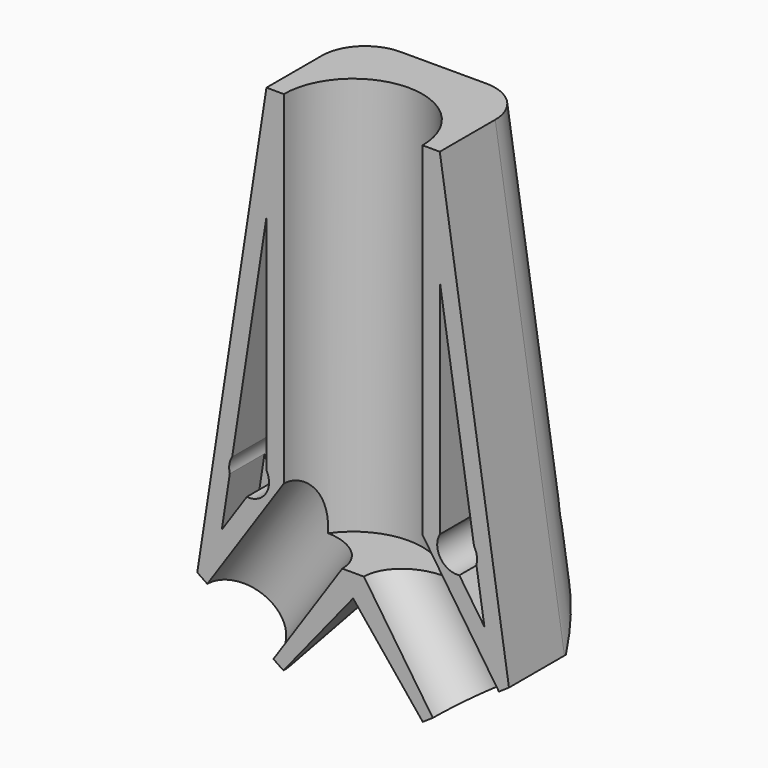
from build123d import *

# Parameters (mm, degrees)
F0_R          = 2.3
F1_DEPTH      = 13
F3_DEPTH      = 46
F6_DEPTH      = 52.2
F8_DEPTH      = 25
F10_DEPTH     = 25
F11_T1_DEPTH  = 69.4664340584
F11_T3_DEPTH  = 69.4664340584
F11_T8_DEPTH  = 31.9524083705
F11_T13_DEPTH = 31.9524083705
F11_T19_DEPTH = 31.9524083705
F11_T23_DEPTH = 31.9524083705
F15_DEPTH     = 5
F16_DEPTH     = 5
F18_R         = 3.2
F19_DEPTH     = 28


# Not quite as in the source:
# - a fillet or chamfer that OpenCascade refuses, or shapes differently, is made with other operations: its cross-section is extruded or revolved along the edge and cut away or added
# - a feature names something its author has since deleted; it is built from what else it names


with BuildPart() as f1:
    # F0 (on Front) → F1 (new body)
    with BuildSketch(Plane.XZ):
        Polygon((10, 40), (-10, 40), (-17.9806351662, -11.8325809017), (-8.0368565166, -18.5498173996), (0, -8.6111112242), (8.0368565166, -18.5498173996), (17.9806351662, -11.8325809017), align=None)
        with Locations((-12, 0)):
            Circle(F0_R, mode=Mode.SUBTRACT)
        with Locations((12, 0)):
            Circle(F0_R, mode=Mode.SUBTRACT)
    extrude(amount=-F1_DEPTH)

    # F2 (on face) → F3 (cut)
    with BuildSketch(Plane.XY.offset(40)):
        with BuildLine():
            Line((-8, 0), (8, 0))
            ThreePointArc((8, 0), (0, 8), (-8, 0))
        make_face()
    extrude(amount=-F3_DEPTH, mode=Mode.SUBTRACT)

    # F5 (on offset) → F6 (cut)
    with BuildSketch(Plane.YZ.offset(25)):
        Polygon((13, -3.9485500787), (4.1381944902, -18.5498173996), (13, -18.5498173996), align=None)
    extrude(amount=-F6_DEPTH, mode=Mode.SUBTRACT)

    # F7 (on face) → F8 (cut)
    with BuildSketch(Plane(origin=(-11.122658813, 0, -16.4652915326), x_dir=(0.8286482208, 0, -0.5597697082), z_dir=(-0.5597697082, 0, -0.8286482208))):
        with BuildLine():
            ThreePointArc((-6.8761009811, 0), (-2.2761009811, -4.6), (2.3238990189, 0))
            Line((2.3238990189, 0), (-6.8761009811, 0))
        make_face()
    extrude(amount=-F8_DEPTH, mode=Mode.SUBTRACT)

    # F9 (on face) → F10 (cut)
    with BuildSketch(Plane(origin=(11.122658813, 0, -16.4652915326), x_dir=(0.8286482208, 0, 0.5597697082), z_dir=(0.5597697082, 0, -0.8286482208))):
        with BuildLine():
            ThreePointArc((-2.3238990189, 0), (2.2761009811, -4.6), (6.8761009811, 0))
            Line((6.8761009811, 0), (-2.3238990189, 0))
        make_face()
    extrude(amount=-F10_DEPTH, mode=Mode.SUBTRACT)

    # F11: fillet of radius 5 on 4 edges, made by hand

    # F11_s2 → F11_t1 (cut)
    with BuildSketch(Plane(origin=(7.6867833124, 0, 49.9240736631), x_dir=(0, 1, 0), z_dir=(-0.152176248, 0, -0.9883533728))):
        with BuildLine():
            ThreePointArc((13, -10.9705836466), (11.5355339059, -14.5061175525), (8, -15.9705836466))
            Line((8, -15.9705836466), (13, -15.9705836466))
            Line((13, -15.9705836466), (13, -10.9705836466))
        make_face()
    extrude(amount=F11_T1_DEPTH, mode=Mode.SUBTRACT)

    # F11_s4 → F11_t3 (cut)
    with BuildSketch(Plane(origin=(2.8843579817, 0, -18.733310736), x_dir=(0, 1, 0), z_dir=(-0.152176248, 0, 0.9883533728))):
        with BuildLine():
            ThreePointArc((8, -15.9705836466), (11.5355339059, -14.5061175525), (13, -10.9705836466))
            Line((13, -10.9705836466), (13, -15.9705836466))
            Line((13, -15.9705836466), (8, -15.9705836466))
        make_face()
    extrude(amount=F11_T3_DEPTH, mode=Mode.SUBTRACT)


with BuildPart() as f11_tool6:
    # F11_s7 → F11_t8 (new body)
    with BuildSketch(Plane(origin=(4.0911710208, 3.0705977915, 5.0593097692), x_dir=(0.6002776597, -0.7997916799, 0), z_dir=(-0.5686414, -0.4267895471, -0.7032052622))):
        with BuildLine():
            ThreePointArc((-10.7347001393, -7.9787789452), (-7.9821654916, -9.2854915519), (-4.9822833283, -8.7519638303))
            Line((-4.9822833283, -8.7519638303), (-8.1340389445, -10.4154145762))
            Line((-8.1340389445, -10.4154145762), (-10.7347001393, -7.9787789452))
        make_face()
    extrude(amount=F11_T8_DEPTH)

    split(bisect_by=Plane(origin=(-4.2102294585, 0, -3.404568911), x_dir=(0, 1, 0), z_dir=(-0.7775800359, 0, -0.6287839754)), keep=Keep.TOP)


with BuildPart() as f1_1:
    add(f1.part)

    # F11_t5: cut F11_tool6
    add(f11_tool6.part, mode=Mode.SUBTRACT)


with BuildPart() as f11_tool11:
    # F11_s12 → F11_t13 (new body)
    with BuildSketch(Plane(origin=(14.0782912081, -10.566356105, -17.4097919354), x_dir=(-0.6002776597, -0.7997916799, 0), z_dir=(-0.5686414, 0.4267895471, 0.7032052622))):
        with BuildLine():
            ThreePointArc((-10.7347001393, -7.9787789452), (-7.9821654916, -9.2854915519), (-4.9822833283, -8.7519638303))
            Line((-4.9822833283, -8.7519638303), (-8.1340389445, -10.4154145762))
            Line((-8.1340389445, -10.4154145762), (-10.7347001393, -7.9787789452))
        make_face()
    extrude(amount=F11_T13_DEPTH)

    split(bisect_by=Plane(origin=(4.2102294585, 0, -3.404568911), x_dir=(0, 1, 0), z_dir=(0.7775800359, 0, -0.6287839754)), keep=Keep.TOP)


with BuildPart() as f1_2:
    add(f1_1.part)

    # F11_t10: cut F11_tool11
    add(f11_tool11.part, mode=Mode.SUBTRACT)


with BuildPart() as f11_tool17:
    # F11_s18 → F11_t19 (new body)
    with BuildSketch(Plane(origin=(14.0782912081, -10.566356105, -17.4097919354), x_dir=(-0.6002776597, -0.7997916799, 0), z_dir=(-0.5686414, 0.4267895471, 0.7032052622))):
        with BuildLine():
            ThreePointArc((-10.7347001393, -7.9787789452), (-7.9821654916, -9.2854915519), (-4.9822833283, -8.7519638303))
            Line((-4.9822833283, -8.7519638303), (-8.1340389445, -10.4154145762))
            Line((-8.1340389445, -10.4154145762), (-10.7347001393, -7.9787789452))
        make_face()
    extrude(amount=F11_T19_DEPTH)

    split(bisect_by=Plane(origin=(4.2102294585, 0, -3.404568911), x_dir=(0, 1, 0), z_dir=(-0.7775800359, 0, 0.6287839754)), keep=Keep.TOP)


with BuildPart() as f11_tool21:
    # F11_s22 → F11_t23 (new body)
    with BuildSketch(Plane(origin=(4.0911710208, 3.0705977915, 5.0593097692), x_dir=(0.6002776597, -0.7997916799, 0), z_dir=(-0.5686414, -0.4267895471, -0.7032052622))):
        with BuildLine():
            ThreePointArc((-10.7347001393, -7.9787789452), (-7.9821654916, -9.2854915519), (-4.9822833283, -8.7519638303))
            Line((-4.9822833283, -8.7519638303), (-8.1340389445, -10.4154145762))
            Line((-8.1340389445, -10.4154145762), (-10.7347001393, -7.9787789452))
        make_face()
    extrude(amount=F11_T23_DEPTH)

    split(bisect_by=Plane(origin=(-4.2102294585, 0, -3.404568911), x_dir=(0, 1, 0), z_dir=(0.7775800359, 0, 0.6287839754)), keep=Keep.TOP)


with BuildPart() as f11_tool17_1:
    add(f11_tool17.part)

    # F11_t25: intersect F11_tool21
    add(f11_tool21.part, mode=Mode.INTERSECT)


with BuildPart() as f1_3:
    add(f1_2.part)

    # F11_t15: cut F11_tool17
    add(f11_tool17_1.part, mode=Mode.SUBTRACT)

    # F14 (on face) → F15 (cut)
    with BuildSketch(Plane.XZ):
        Polygon((-15.1459260242, -6.5643846345), (-10, 1.0533238305), (-10, 26.8573445146), align=None)
    extrude(amount=-F15_DEPTH, mode=Mode.SUBTRACT)

    # F12 (on face) → F16 (cut)
    with BuildSketch(Plane.XZ):
        Polygon((15.1459253956, -6.5643830302), (10.0000003771, 26.8573395869), (10.0000003771, 1.0533239459), align=None)
    extrude(amount=-F16_DEPTH, mode=Mode.SUBTRACT)

    # F18 (on offset) → F19 (cut)
    with BuildSketch(Plane(origin=(0, 38, 0), x_dir=(-1, 0, 0), z_dir=(0, 1, 0))):
        with Locations((-12, 0)):
            Circle(F18_R)
        with Locations((12, 0)):
            Circle(F18_R)
    extrude(amount=-F19_DEPTH, mode=Mode.SUBTRACT)


solid = f1_3.part
